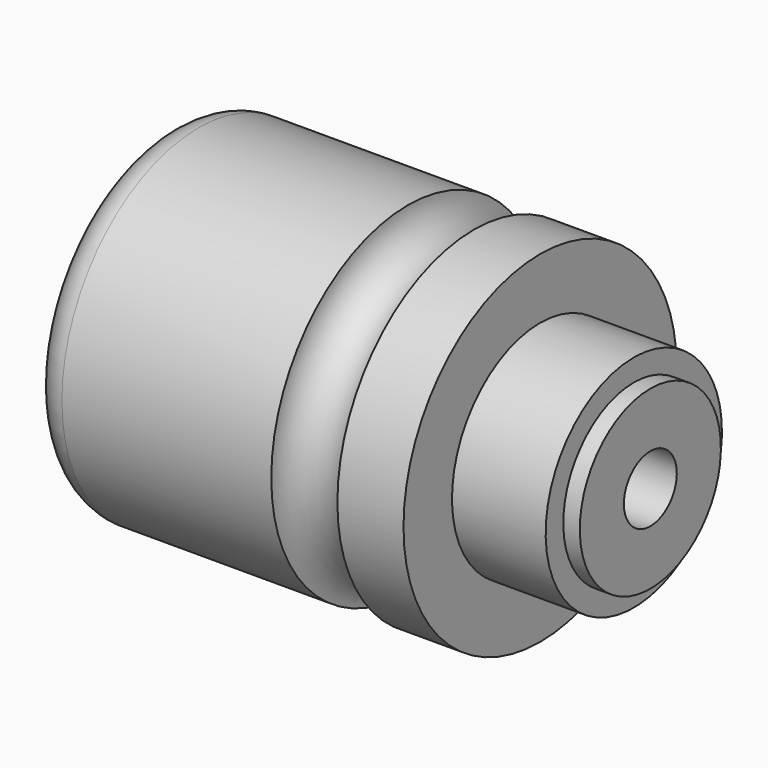
from build123d import *

# Parameters (mm, degrees)
F4_R = 5.99999


# Not quite as in the source:
# - a fillet or chamfer is up to 0.001 mm smaller than in the source, because OpenCascade refuses the exact size


with BuildPart() as f1:
    # F0 (on Front) → F1 (revolve)
    with BuildSketch(Plane.XZ):
        with BuildLine():
            Line((0, 31), (0, 0))
            Line((0, 0), (88, 0))
            Line((88, 0), (88, 16))
            Line((88, 16), (85, 16))
            Line((85, 16), (85, 20))
            Line((85, 20), (68, 20))
            Line((68, 20), (68, 31))
            Line((68, 31), (56, 31))
            ThreePointArc((56, 31), (50, 25), (44, 31))
            Line((44, 31), (0, 31))
        make_face()
    revolve(axis=Axis((50, 0, 0), (1, 0, 0)))

    # F2 (on Front) → F3 (revolve, cut)
    with BuildSketch(Plane.XZ):
        Polygon((0, 25), (0, 0), (88, 0), (88, 6), (30, 6), (30, 16), (22, 16), (22, 20.5), (15, 20.5), (15, 12.5), (12, 12.5), (12, 16), (1.5, 16), (1.5, 25), align=None)
    revolve(axis=Axis((-8.7147882535, 0, 0), (-1, 0, 0)), mode=Mode.SUBTRACT)

    # F4 (radius 6 in the source; OpenCascade refuses exactly that, so slightly less here)
    f4_edges = [f1.edges().sort_by_distance(p)[0] for p in [
        (0, 0, -31),
    ]]
    fillet(f4_edges, radius=F4_R)


solid = f1.part
